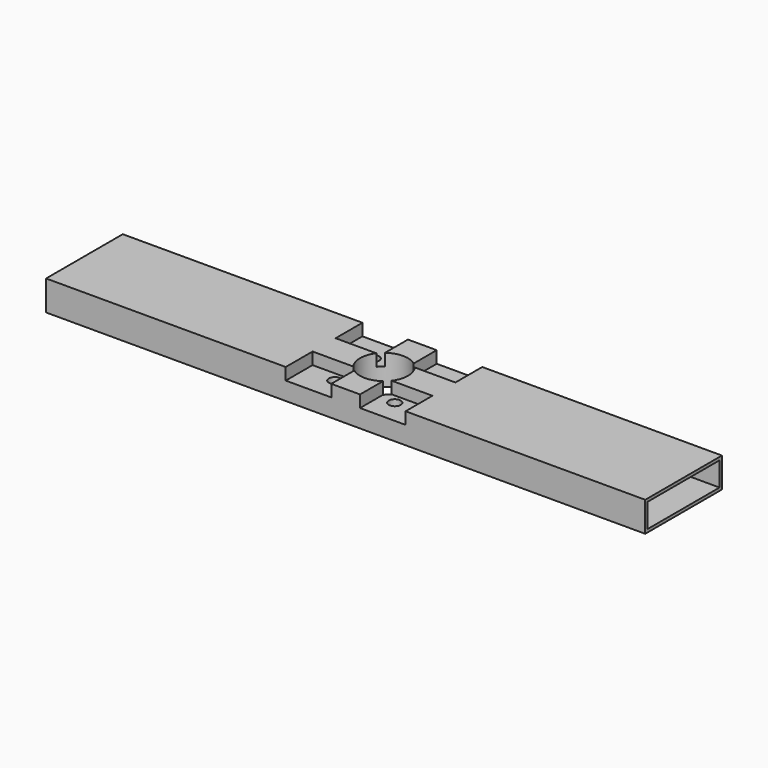
from build123d import *

# Parameters (mm, degrees)
F0_W         = 500
F0_H         = 80
F1_DEPTH     = 25
F3_D         = 40
F3_DEPTH     = 25
F3_TIP       = 12.0172123806
F4_D         = 10
F4_DEPTH     = 25
F4_TIP       = 3.0043030951
F2_W         = 38
F2_H         = 28
F5_DEPTH     = 10
F6_T         = 2.5
F6_T3_DEPTH  = 15
F6_T5_DEPTH  = 33
F6_T7_DEPTH  = 29
F6_T9_DEPTH  = 39
F6_T11_DEPTH = 39
F6_T13_DEPTH = 33
F6_T15_DEPTH = 29


# Not quite as in the source:
# - a shell that OpenCascade refuses in one call is made with other operations: the cavity is built on its own and cut out


with BuildPart() as f1:
    # F0 (on Top) → F1 (new body)
    with BuildSketch(Plane.XY):
        Rectangle(F0_W, F0_H)
    extrude(amount=F1_DEPTH)

    # F3
    with Locations(Plane.XY.offset(25)):
        with Locations((0, 0)):
            Hole(F3_D / 2, depth=F3_DEPTH)
            with Locations((0, 0, -(F3_DEPTH + F3_TIP / 2))):  # 118° drill point
                Cone(0, F3_D / 2, F3_TIP, mode=Mode.SUBTRACT)

    # F4
    with Locations(Plane.XY.offset(25)):
        with Locations((-25, 20), (25, 20), (25, -20), (-25, -20)):
            Hole(F4_D / 2, depth=F4_DEPTH)
            with Locations((0, 0, -(F4_DEPTH + F4_TIP / 2))):  # 118° drill point
                Cone(0, F4_D / 2, F4_TIP, mode=Mode.SUBTRACT)

    # F2 (on face) → F5 (cut)
    with BuildSketch(Plane.XY.offset(25)):
        with Locations((-31, -26)):
            Rectangle(F2_W, F2_H)
        with Locations((-31, 26)):
            Rectangle(F2_W, F2_H)
        with Locations((31, 26)):
            Rectangle(F2_W, F2_H)
        with Locations((31, -26)):
            Rectangle(F2_W, F2_H)
    extrude(amount=-F5_DEPTH, mode=Mode.SUBTRACT)

    # F6: shell of thickness 2.5, made by hand


with BuildPart() as f6_core1:
    # F6_t2: copy of F1
    add(f1.part)

    # the walls: a layer under each face that stays
    f6_faces = [f6_core1.faces().sort_by_distance(p)[0] for p in [
        (0, 40, 12.5),
        (-166.6666666667, -26.6666666667, 0),
        (-133, 0, 25),
        (-50, 26, 20),
        (-31, 26, 15),
        (-12, 28, 20),
        (0, 28, 25),
        (12, 28, 20),
        (31, 26, 15),
        (50, 26, 20),
        (133, 0, 25),
        (0, -40, 12.5),
        (-30, -20, 7.5),
        (20, -20, 7.5),
        (-30, 20, 7.5),
        (-20, 0, 12.5),
        (20, 20, 7.5),
        (-33, 12, 20),
        (-33, -12, 20),
        (-50, -26, 20),
        (33, 12, 20),
        (50, -26, 20),
        (33, -12, 20),
        (31, -26, 15),
        (12, -28, 20),
        (0, -28, 25),
        (-12, -28, 20),
        (-31, -26, 15),
    ]]
    thicken(f6_faces, amount=-F6_T, mode=Mode.SUBTRACT)

    # F6_s4 → F6_t3 (cut)
    with BuildSketch(Plane.XY.offset(12.5)):
        Polygon((-49.975, 12.025), (-52.5, 12), (-52.5, 9.5), (-50, 9.5), align=None)
        Polygon((49.975, 12.025), (52.5, 12), (52.5, 9.5), (50, 9.5), align=None)
        Polygon((-49.975, -12.025), (-50, -9.5), (-52.5, -9.5), (-52.5, -12), align=None)
        Polygon((49.975, -12.025), (52.5, -12), (52.5, -9.5), (50, -9.5), align=None)
    extrude(amount=F6_T3_DEPTH, mode=Mode.SUBTRACT)

    # F6_s6 → F6_t5 (cut)
    with BuildSketch(Plane.XZ.offset(-42.5)):
        Polygon((-49.975, 15.025), (-52.5, 15), (-52.5, 12.5), (-50, 12.5), align=None)
        Polygon((49.975, 15.025), (50, 12.5), (52.5, 12.5), (52.5, 15), align=None)
    extrude(amount=F6_T5_DEPTH, mode=Mode.SUBTRACT)

    # F6_s8 → F6_t7 (cut)
    with BuildSketch(Plane.XZ.offset(-42.5)):
        Polygon((-12.025, 15.025), (-12, 12.5), (-9.5, 12.5), (-9.5, 15), align=None)
        Polygon((12.025, 15.025), (9.5, 15), (9.5, 12.5), (12, 12.5), align=None)
    extrude(amount=F6_T7_DEPTH, mode=Mode.SUBTRACT)

    # F6_s10 → F6_t9 (cut)
    with BuildSketch(Plane.YZ.offset(-52.5)):
        Polygon((12.025, 15.025), (12, 12.5), (9.5, 12.5), (9.5, 15), align=None)
        Polygon((-12.025, 15.025), (-9.5, 15), (-9.5, 12.5), (-12, 12.5), align=None)
    extrude(amount=F6_T9_DEPTH, mode=Mode.SUBTRACT)

    # F6_s12 → F6_t11 (cut)
    with BuildSketch(Plane.YZ.offset(13.5)):
        Polygon((12.025, 15.025), (12, 12.5), (9.5, 12.5), (9.5, 15), align=None)
        Polygon((-12.025, 15.025), (-9.5, 15), (-9.5, 12.5), (-12, 12.5), align=None)
    extrude(amount=F6_T11_DEPTH, mode=Mode.SUBTRACT)

    # F6_s14 → F6_t13 (cut)
    with BuildSketch(Plane.XZ.offset(9.5)):
        Polygon((-49.975, 15.025), (-52.5, 15), (-52.5, 12.5), (-50, 12.5), align=None)
        Polygon((49.975, 15.025), (52.5, 15), (52.5, 12.5), (50, 12.5), align=None)
    extrude(amount=F6_T13_DEPTH, mode=Mode.SUBTRACT)

    # F6_s16 → F6_t15 (cut)
    with BuildSketch(Plane.XZ.offset(13.5)):
        Polygon((12.025, 15.025), (12, 12.5), (9.5, 12.5), (9.5, 15), align=None)
        Polygon((-12.025, 15.025), (-9.5, 15), (-9.5, 12.5), (-12, 12.5), align=None)
    extrude(amount=F6_T15_DEPTH, mode=Mode.SUBTRACT)


with BuildPart() as f1_1:
    add(f1.part)

    # what is left inside the walls is the cavity
    f6_cavity = [f6_core1.part.solids().sort_by_distance(p)[0] for p in [
        (-125, 12.5, 2.525),
    ]]
    add(f6_cavity, mode=Mode.SUBTRACT)


solid = f1_1.part
